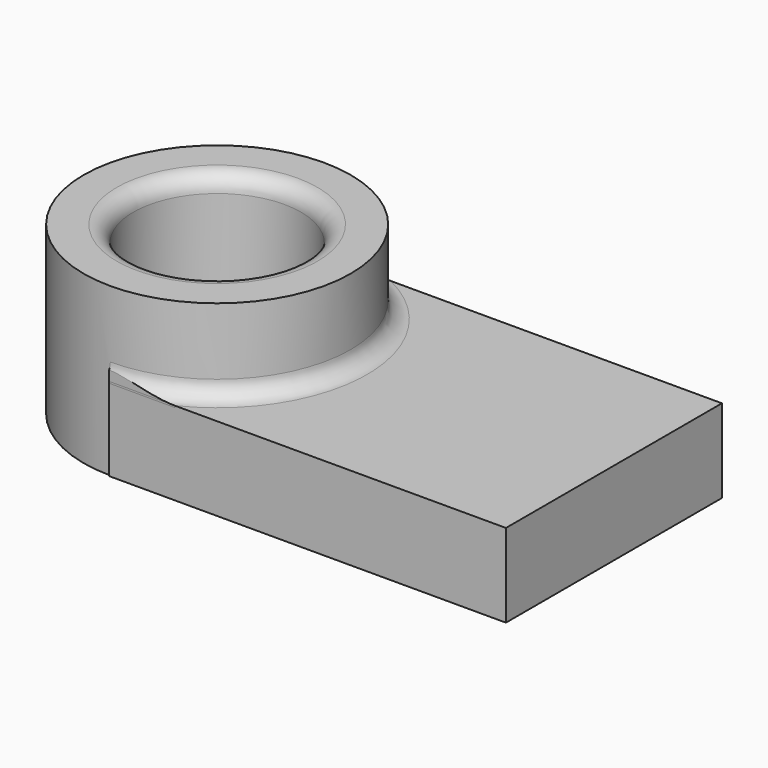
from build123d import *

# Parameters (mm, degrees)
F1_DEPTH    = 25.4
F2_DEPTH    = 50.8
F4_T4_ANGLE = 180


# Not quite as in the source:
# - a fillet or chamfer that OpenCascade refuses, or shapes differently, is made with other operations: its cross-section is extruded or revolved along the edge and cut away or added
# - a feature of the source that left no trace in its solid (it failed there, or was rolled back) is left out


with BuildPart() as f1:
    # F0 (on Top) → F1 (new body)
    with BuildSketch(Plane.XY):
        with BuildLine():
            Line((60.4218803346, 41.1163568497), (-60.4218803346, 41.1163568497))
            Line((-60.4218803346, 41.1163568497), (-60.4218803346, 40.6873208554))
            ThreePointArc((-60.4218803346, 40.6873208554), (-31.6515998495, 28.7702804852), (-19.7345594792, 0))
            ThreePointArc((-19.7345594792, 0), (-31.6515998495, -28.7702804852), (-60.4218803346, -40.6873208554))
            Line((-60.4218803346, -40.6873208554), (-60.4218803346, -41.1163568497))
            Line((-60.4218803346, -41.1163568497), (60.4218803346, -41.1163568497))
            Line((60.4218803346, -41.1163568497), (60.4218803346, 41.1163568497))
        make_face()
        with BuildLine():
            ThreePointArc((-19.7345594792, 0), (-31.6515998495, 28.7702804852), (-60.4218803346, 40.6873208554))
            Line((-60.4218803346, 40.6873208554), (-60.4218803346, 25.5206269771))
            ThreePointArc((-60.4218803346, 25.5206269771), (-42.376071939, 18.0458083957), (-34.9012533575, 0))
            ThreePointArc((-34.9012533575, 0), (-42.376071939, -18.0458083957), (-60.4218803346, -25.5206269771))
            Line((-60.4218803346, -25.5206269771), (-60.4218803346, -40.6873208554))
            ThreePointArc((-60.4218803346, -40.6873208554), (-31.6515998495, -28.7702804852), (-19.7345594792, 0))
        make_face()
        with BuildLine():
            Line((-60.4218803346, 25.5206269771), (-60.4218803346, 40.6873208554))
            ThreePointArc((-60.4218803346, 40.6873208554), (-101.10920119, 0), (-60.4218803346, -40.6873208554))
            Line((-60.4218803346, -40.6873208554), (-60.4218803346, -25.5206269771))
            ThreePointArc((-60.4218803346, -25.5206269771), (-85.9425073118, 0), (-60.4218803346, 25.5206269771))
        make_face()
    extrude(amount=F1_DEPTH)

    # F0 (on Top) → F2 (join)
    with BuildSketch(Plane.XY):
        with BuildLine():
            Line((-60.4218803346, 25.5206269771), (-60.4218803346, 40.6873208554))
            ThreePointArc((-60.4218803346, 40.6873208554), (-101.10920119, 0), (-60.4218803346, -40.6873208554))
            Line((-60.4218803346, -40.6873208554), (-60.4218803346, -25.5206269771))
            ThreePointArc((-60.4218803346, -25.5206269771), (-85.9425073118, 0), (-60.4218803346, 25.5206269771))
        make_face()
        with BuildLine():
            ThreePointArc((-19.7345594792, 0), (-31.6515998495, 28.7702804852), (-60.4218803346, 40.6873208554))
            Line((-60.4218803346, 40.6873208554), (-60.4218803346, 25.5206269771))
            ThreePointArc((-60.4218803346, 25.5206269771), (-42.376071939, 18.0458083957), (-34.9012533575, 0))
            ThreePointArc((-34.9012533575, 0), (-42.376071939, -18.0458083957), (-60.4218803346, -25.5206269771))
            Line((-60.4218803346, -25.5206269771), (-60.4218803346, -40.6873208554))
            ThreePointArc((-60.4218803346, -40.6873208554), (-31.6515998495, -28.7702804852), (-19.7345594792, 0))
        make_face()
    extrude(amount=F2_DEPTH)

    # F4: fillet of radius 5.08 on 6 edges, made by hand


with BuildPart() as f4_tool2:
    # F4_s3 → F4_t4 (revolve)
    with BuildSketch(Plane.YZ.offset(-60.4218803346)):
        with BuildLine():
            ThreePointArc((45.7682865408, 25.3996), (42.175218407, 26.8878975516), (40.6869208554, 30.4809656854))
            Line((40.6869208554, 30.4809656854), (40.1787842868, 30.4809656854))
            ThreePointArc((40.1787842868, 30.4809656854), (40.1791842868, 27.9404828427), (40.1791842868, 25.4))
            Line((40.1791842868, 25.4), (40.6873208554, 24.8918634315))
            ThreePointArc((40.6873208554, 24.8918634315), (43.2278036981, 24.8918634315), (45.7682865408, 24.8914634315))
            Line((45.7682865408, 24.8914634315), (45.7682865408, 25.3996))
        make_face()
    revolve(axis=Axis((-60.4218803346, 0, 25.4), (0, 0, -1)), revolution_arc=F4_T4_ANGLE)

    split(bisect_by=Plane.XZ.offset(-41.1163568497), keep=Keep.TOP)

    split(bisect_by=Plane.XZ.offset(41.1163568497), keep=Keep.BOTTOM)


with BuildPart() as f1_1:
    add(f1.part)

    # F4_t1: union F4_tool2
    add(f4_tool2.part)

    # F4_s7 → F4_t8 (revolve, cut)
    with BuildSketch(Plane.YZ.offset(-60.4218803346)):
        with BuildLine():
            ThreePointArc((30.6015926626, 50.8004), (27.0085245287, 49.3121024484), (25.5202269771, 45.7190343146))
            Line((25.5202269771, 45.7190343146), (25.0120904086, 45.7190343146))
            ThreePointArc((25.0120904086, 45.7190343146), (25.0124904086, 48.2595171573), (25.0124904086, 50.8))
            Line((25.0124904086, 50.8), (25.5206269771, 51.3081365685))
            ThreePointArc((25.5206269771, 51.3081365685), (28.0611098198, 51.3081365685), (30.6015926626, 51.3085365685))
            Line((30.6015926626, 51.3085365685), (30.6015926626, 50.8004))
        make_face()
    revolve(axis=Axis((-60.4218803346, 0, 50.8), (0, 0, -1)), mode=Mode.SUBTRACT)

    # F4_s9 → F4_t10 (revolve, cut)
    with BuildSketch(Plane.YZ.offset(-60.4218803346)):
        with BuildLine():
            ThreePointArc((-25.5202269771, 5.0809656854), (-27.0085245287, 1.4878975516), (-30.6015926626, -0.0004))
            Line((-30.6015926626, -0.0004), (-30.6015926626, -0.5085365685))
            ThreePointArc((-30.6015926626, -0.5085365685), (-28.0611098198, -0.5081365685), (-25.5206269771, -0.5081365685))
            Line((-25.5206269771, -0.5081365685), (-25.0124904086, 0))
            ThreePointArc((-25.0124904086, 0), (-25.0124904086, 2.5404828427), (-25.0120904086, 5.0809656854))
            Line((-25.0120904086, 5.0809656854), (-25.5202269771, 5.0809656854))
        make_face()
    revolve(axis=Axis((-60.4218803346, 0, 0), (0, 0, 1)), mode=Mode.SUBTRACT)


solid = f1_1.part
